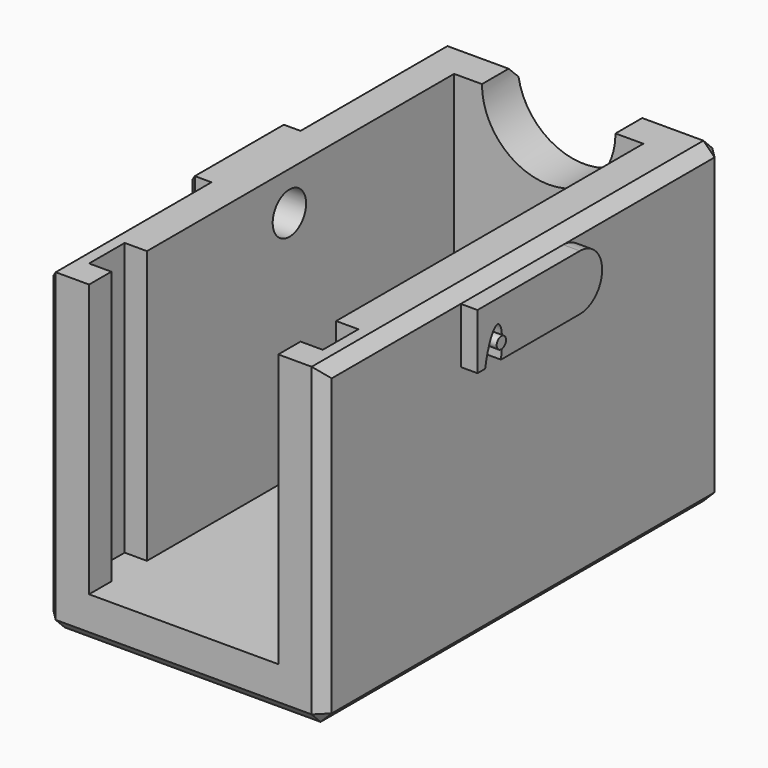
from build123d import *

# Parameters (mm, degrees)
F0_W      = 50
F0_H      = 90
F1_DEPTH  = 8
F3_DEPTH  = 49
F4_R      = 3.75
F5_DEPTH  = 25
F7_DEPTH  = 50
F9_START  = -25
F8_W      = 20
F8_H      = 14
F9_DEPTH  = 3
F11_START = 25
F11_DEPTH = 3
F13_START = 25
F12_R     = 1.0510148408
F13_DEPTH = 4
F14_SIZE  = 1.99999


# Not quite as in the source:
# - a fillet or chamfer is up to 0.001 mm smaller than in the source, because OpenCascade refuses the exact size


with BuildPart() as f1:
    # F0 (on Top) → F1 (new body)
    with BuildSketch(Plane.XY):
        Rectangle(F0_W, F0_H)
    extrude(amount=-F1_DEPTH)

    # F2 (on Top) → F3 (join)
    with BuildSketch(Plane.XY):
        Polygon((-17, 45), (-25, 45), (-25, 37), (-25, -45), (-17, -45), (-17, -40), (-21, -40), (-21, -32), (-17, -32), (-17, 37), (17, 37), (17, -32), (21, -32), (21, -40), (17, -40), (17, -45), (25, -45), (25, 37), (25, 45), (17, 45), align=None)
    extrude(amount=F3_DEPTH)

    # F4 (on Right) → F5 (cut, symmetric)
    with BuildSketch(Plane.YZ):
        with Locations((0, 42)):
            Circle(F4_R)
    extrude(amount=F5_DEPTH, both=True, mode=Mode.SUBTRACT)

    # F6 (on Front) → F7 (cut)
    with BuildSketch(Plane.XZ):
        with BuildLine():
            ThreePointArc((-12, 49), (0, 37), (12, 49))
            Line((12, 49), (-12, 49))
        make_face()
    extrude(amount=-F7_DEPTH, mode=Mode.SUBTRACT)

    # F8 (on Right) → F9 (join)
    with BuildSketch(Plane.YZ.offset(F9_START)):
        with Locations((0, 42)):
            Rectangle(F8_W, F8_H)
    extrude(amount=-F9_DEPTH)

    # F10 (on Right) → F11 (join)
    with BuildSketch(Plane.YZ.offset(F11_START)):
        with BuildLine():
            ThreePointArc((14, 42), (12.5355339059, 45.5355339059), (9, 47))
            Line((9, 47), (-14, 47))
            Line((-14, 47), (-14, 37))
            Line((-14, 37), (-12.275, 37))
            add(Edge.make_bspline(
                [(-8.722, 37), (-7.7358158763, 42.9104981706), (-9.5123158763, 42.9104981706), (-11.2888158763, 42.9104981706), (-12.275, 37)],
                knots=[4.765680137, 4.765680137, 4.765680137, 6.3364764638, 6.3364764638, 7.9072727906, 7.9072727906, 7.9072727906], degree=2, weights=[1, 0.7071067812, 1, 0.7071067812, 1]))
            Line((-8.722, 37), (9, 37))
            ThreePointArc((9, 37), (12.5355339059, 38.4644660941), (14, 42))
        make_face()
    extrude(amount=F11_DEPTH)

    # F12 (on Right) → F13 (join)
    with BuildSketch(Plane.YZ.offset(F13_START)):
        with Locations((-9.8914606497, 40.4975526035)):
            Circle(F12_R)
    extrude(amount=F13_DEPTH)

    # F14 (size 2 in the source; OpenCascade refuses exactly that, so slightly less here)
    f14_edges = [f1.edges().sort_by_distance(p)[0] for p in [
        (25, 0, -8),
        (25, -45, 20.5),
        (0, -45, -8),
        (-25, -45, 20.5),
        (-25, 0, -8),
        (-25, 45, 20.5),
        (25, 45, 20.5),
        (0, 45, -8),
        (-28, 0, 49),
        (-18.5, 45, 49),
        (18.5, 45, 49),
        (25, 0, 49),
        (-25, 27.5, 49),
        (-25, -27.5, 49),
        (-28, 10, 42),
        (-28, 0, 35),
        (-28, -10, 42),
    ]]
    chamfer(f14_edges, length=F14_SIZE)


solid = f1.part
